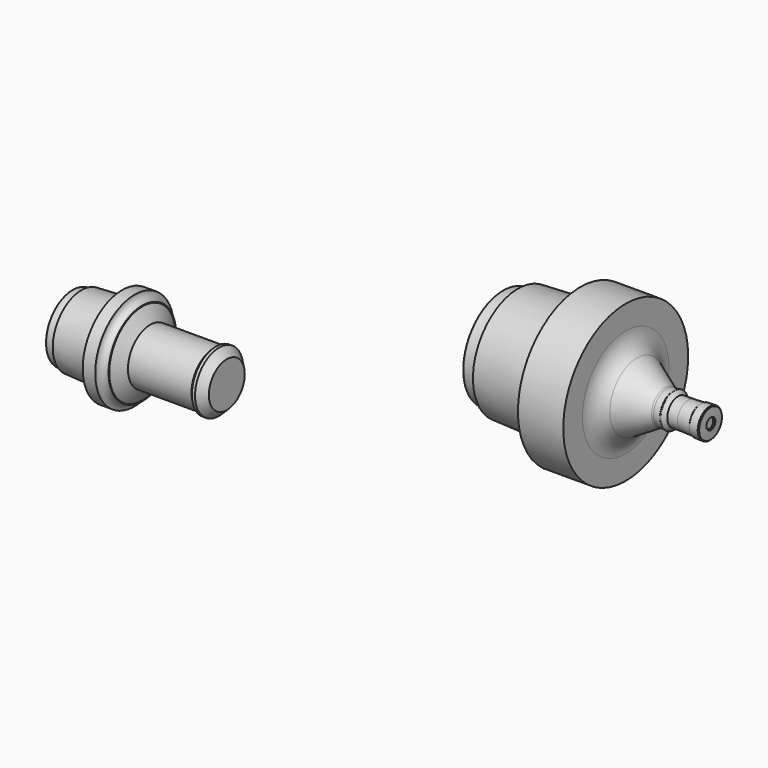
from build123d import *


# Not quite as in the source:
# - ends of sketch curves that miss each other by under 0.0002 mm in the source are joined


with BuildPart() as f1:
    # F0 (on Top) → F1 (revolve)
    with BuildSketch(Plane.XY):
        with BuildLine():
            Line((210.527722, 136.986687), (210.527722, 152.345305))
            Line((210.527722, 152.345305), (181.527722, 152.345305))
            Line((181.527722, 152.345305), (181.527722, 140.345278))
            Line((181.527722, 140.345278), (141.519722, 138.345305))
            Line((141.519722, 138.345305), (141.527722, 134.557305))
            Line((141.527722, 134.557305), (132.613144, 134.42734))
            ThreePointArc((132.613144, 134.42734), (131.9154797673, 134.1293797589), (131.627722, 133.427446))
            Line((131.627722, 133.427446), (131.627722, 102.345305))
            Line((131.627722, 102.345305), (264.134658, 102.345305))
            Line((264.134658, 102.345305), (264.134658, 105.413028))
            Line((264.134658, 105.413028), (264.579927, 105.429279))
            Line((264.579927, 105.429279), (265.074113, 105.961073))
            Line((265.074113, 105.961073), (264.87187, 111.450896))
            Line((264.87187, 111.450896), (264.339882, 111.945237))
            Line((264.339882, 111.945237), (258.849853, 111.744866))
            Line((258.849853, 111.744866), (258.443342, 111.307419))
            Line((258.443342, 111.307419), (250.622956, 111.034622))
            Line((250.622956, 111.034622), (244.101081, 111.034622))
            Line((244.101081, 111.034622), (241.848977, 113.286726))
            ThreePointArc((241.848977, 113.286726), (241.566134, 113.403883), (241.2832912875, 113.2867257125))
            Line((241.2832912875, 113.2867257125), (241.031187, 113.034622))
            Line((241.031187, 113.034622), (236.821241, 113.034622))
            ThreePointArc((236.821241, 113.034622), (236.2867644086, 113.107361049), (235.7911651362, 113.3202872267))
            Line((235.7911651362, 113.3202872267), (217.802151, 124.129177))
            ThreePointArc((217.802151, 124.129177), (212.4723866491, 129.6003334426), (210.527722, 136.986687))
        make_face()
    revolve(axis=Axis((197.88119, 102.345305, 0), (-1, 0, 0)))


with BuildPart() as f3:
    # F2 (on Top) → F3 (revolve)
    with BuildSketch(Plane.XY):
        with BuildLine():
            Line((-49.538447, 4.765), (-49.538447, -15.75))
            Line((-49.538447, -15.75), (49.538447, -15.75))
            Line((49.538447, -15.75), (49.538447, -1.37172))
            Line((49.538447, -1.37172), (44.618447, 3.529558))
            Line((44.618447, 3.529558), (42.618447, 3.529558))
            Line((42.618447, 3.529558), (41.151866, 2.068558))
            Line((41.151866, 2.068558), (0.473786, 2.068558))
            Line((0.473786, 2.068558), (-4.538447, 10.75))
            Line((-4.538447, 10.75), (-4.538447, 11.25))
            Line((-4.538447, 11.25), (-5.038447, 11.25))
            ThreePointArc((-5.038447, 11.25), (-8.2204275153, 12.5680194847), (-9.538447, 15.75))
            Line((-9.538447, 15.75), (-17.538447, 15.75))
            Line((-17.538447, 15.75), (-17.538447, 8.565))
            Line((-17.538447, 8.565), (-43.538447, 7.265))
            Line((-43.538447, 7.265), (-43.538447, 5.765))
            Line((-43.538447, 5.765), (-48.538447, 5.765))
            ThreePointArc((-48.538447, 5.765), (-49.2455537812, 5.4721067812), (-49.538447, 4.765))
        make_face()
    revolve(axis=Axis((0, -15.75, 0), (1, 0, 0)))


solid = Compound([f1.part, f3.part])
